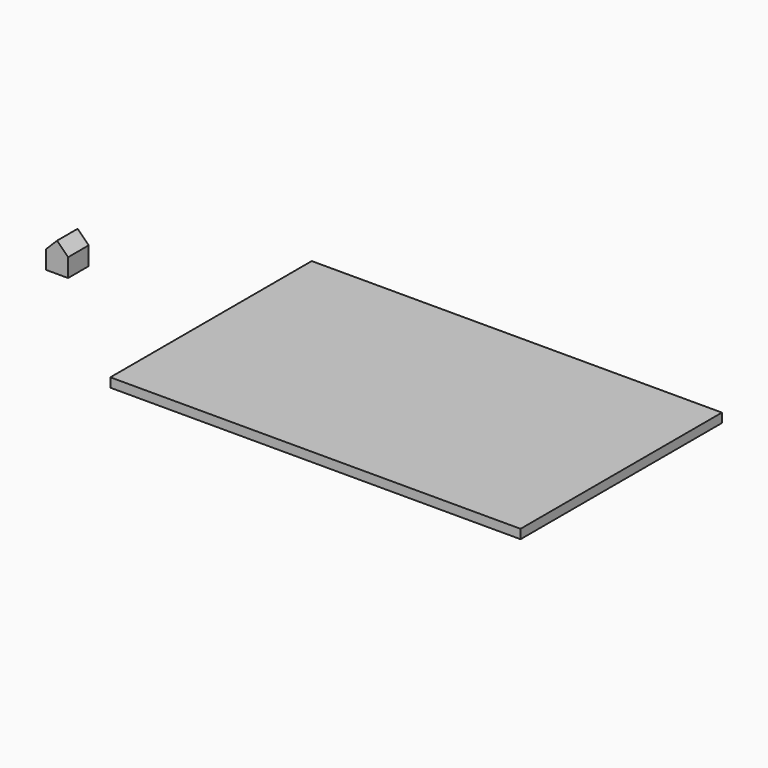
from build123d import *

# Parameters (mm, degrees)
F0_W     = 1117.6
F0_H     = 685.8
F1_DEPTH = 25
F2_W     = 60
F2_H     = 70
F3_DEPTH = 80
F4_SIZE  = 29.99999


# Not quite as in the source:
# - a fillet or chamfer is up to 0.001 mm smaller than in the source, because OpenCascade refuses the exact size


with BuildPart() as f1:
    # F0 (on Top) → F1 (new body)
    with BuildSketch(Plane.XY):
        with Locations((-15.9892961383, -43.4064045523)):
            Rectangle(F0_W, F0_H)
    extrude(amount=F1_DEPTH)


with BuildPart() as f3:
    # F2 (on Top) → F3 (new body)
    with BuildSketch(Plane.XY):
        with Locations((-990.582793951, -12.9387065261)):
            Rectangle(F2_W, F2_H)
    extrude(amount=F3_DEPTH)

    # F4 (size 30 in the source; OpenCascade refuses exactly that, so slightly less here)
    f4_edges = [f3.edges().sort_by_distance(p)[0] for p in [
        (-1020.582794, -12.938707, 80),
        (-960.582794, -12.938707, 80),
    ]]
    chamfer(f4_edges, length=F4_SIZE)


solid = Compound([f1.part, f3.part])
